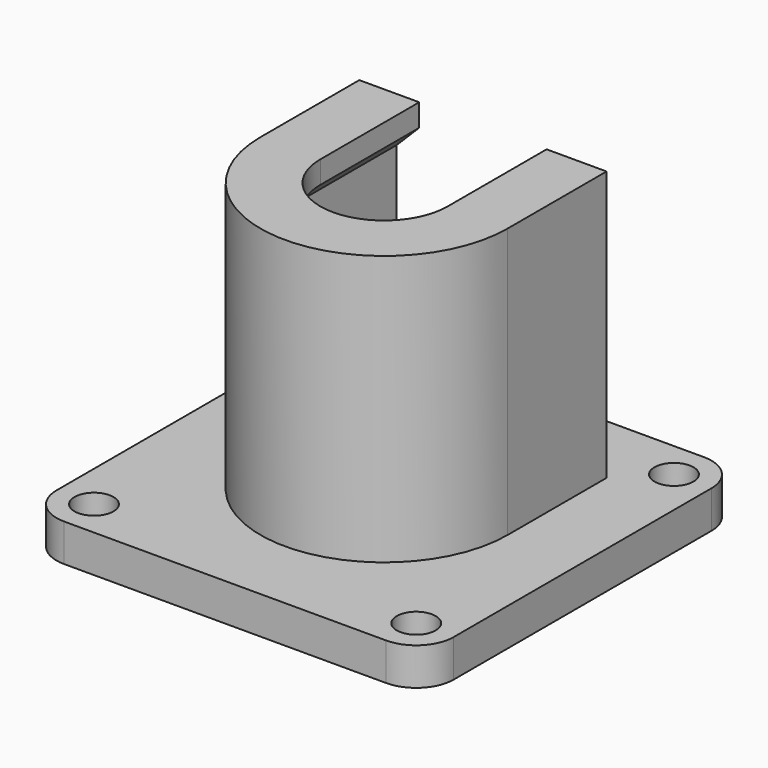
from build123d import *

# Parameters (mm, degrees)
F0_R     = 2.6
F1_DEPTH = 5
F3_DEPTH = 36
F6_DEPTH = 3
F9_DEPTH = 3
F10_SIZE = 2.99999


# Not quite as in the source:
# - a fillet or chamfer is up to 0.001 mm smaller than in the source, because OpenCascade refuses the exact size


with BuildPart() as f1:
    # F0 (on Top) → F1 (new body)
    with BuildSketch(Plane.XY):
        with BuildLine():
            Line((21.5, 26.5), (-21.5, 26.5))
            ThreePointArc((-21.5, 26.5), (-17.9644660941, 25.0355339059), (-16.5, 21.5))
            ThreePointArc((-16.5, 21.5), (-21.5, 16.5), (-26.5, 21.5))
            Line((-26.5, 21.5), (-26.5, -21.5))
            ThreePointArc((-26.5, -21.5), (-21.5, -16.5), (-16.5, -21.5))
            ThreePointArc((-16.5, -21.5), (-17.9644660941, -25.0355339059), (-21.5, -26.5))
            Line((-21.5, -26.5), (21.5, -26.5))
            ThreePointArc((21.5, -26.5), (17.9644660941, -17.9644660941), (26.5, -21.5))
            Line((26.5, -21.5), (26.5, 21.5))
            ThreePointArc((26.5, 21.5), (17.9644660941, 17.9644660941), (21.5, 26.5))
        make_face()
        with BuildLine():
            Line((-11.5, 16.5), (-11.5, 0))
            ThreePointArc((-11.5, 0), (0, -11.5), (11.5, 0))
            Line((11.5, 0), (11.5, 16.5))
            Line((11.5, 16.5), (16.5, 16.5))
            Line((16.5, 16.5), (16.5, 0))
            ThreePointArc((16.5, 0), (0, -16.5), (-16.5, 0))
            Line((-16.5, 0), (-16.5, 16.5))
            Line((-16.5, 16.5), (-11.5, 16.5))
        make_face(mode=Mode.SUBTRACT)
        with BuildLine():
            ThreePointArc((11.5, 0), (0, -11.5), (-11.5, 0))
            Line((-11.5, 0), (-11.5, 16.5))
            Line((-11.5, 16.5), (-16.5, 16.5))
            Line((-16.5, 16.5), (-16.5, 0))
            ThreePointArc((-16.5, 0), (0, -16.5), (16.5, 0))
            Line((16.5, 0), (16.5, 16.5))
            Line((16.5, 16.5), (11.5, 16.5))
            Line((11.5, 16.5), (11.5, 0))
        make_face()
        with BuildLine():
            ThreePointArc((-16.5, 21.5), (-17.9644660941, 25.0355339059), (-21.5, 26.5))
            ThreePointArc((-21.5, 26.5), (-25.0355339059, 25.0355339059), (-26.5, 21.5))
            ThreePointArc((-26.5, 21.5), (-21.5, 16.5), (-16.5, 21.5))
        make_face()
        with Locations((-21.5, 21.5)):
            Circle(F0_R, mode=Mode.SUBTRACT)
        with BuildLine():
            ThreePointArc((-16.5, -21.5), (-21.5, -16.5), (-26.5, -21.5))
            ThreePointArc((-26.5, -21.5), (-25.0355339059, -25.0355339059), (-21.5, -26.5))
            ThreePointArc((-21.5, -26.5), (-17.9644660941, -25.0355339059), (-16.5, -21.5))
        make_face()
        with Locations((-21.5, -21.5)):
            Circle(F0_R, mode=Mode.SUBTRACT)
        with BuildLine():
            ThreePointArc((21.5, -26.5), (25.0355339059, -25.0355339059), (26.5, -21.5))
            ThreePointArc((26.5, -21.5), (17.9644660941, -17.9644660941), (21.5, -26.5))
        make_face()
        with Locations((21.5, -21.5)):
            Circle(F0_R, mode=Mode.SUBTRACT)
        with BuildLine():
            ThreePointArc((26.5, 21.5), (25.0355339059, 25.0355339059), (21.5, 26.5))
            ThreePointArc((21.5, 26.5), (17.9644660941, 17.9644660941), (26.5, 21.5))
        make_face()
        with Locations((21.5, 21.5)):
            Circle(F0_R, mode=Mode.SUBTRACT)
    extrude(amount=F1_DEPTH)

    # F2 (on face) → F3 (join)
    with BuildSketch(Plane.XY.offset(5)):
        with BuildLine():
            ThreePointArc((11.5, 0), (0, -11.5), (-11.5, 0))
            Line((-11.5, 0), (-11.5, 16.5))
            Line((-11.5, 16.5), (-16.5, 16.5))
            Line((-16.5, 16.5), (-16.5, 0))
            ThreePointArc((-16.5, 0), (0, -16.5), (16.5, 0))
            Line((16.5, 0), (16.5, 16.5))
            Line((16.5, 16.5), (11.5, 16.5))
            Line((11.5, 16.5), (11.5, 0))
        make_face()
    extrude(amount=F3_DEPTH)

    # F5 (on offset) → F6 (join)
    with BuildSketch(Plane.XY.offset(15)):
        with BuildLine():
            Line((-11.5, 16.5), (-11.5, 0))
            ThreePointArc((-11.5, 0), (0, -11.5), (11.5, 0))
            Line((11.5, 0), (11.5, 16.5))
            Line((11.5, 16.5), (8.5, 16.5))
            Line((8.5, 16.5), (8.5, 0))
            ThreePointArc((8.5, 0), (0, -8.5), (-8.5, 0))
            Line((-8.5, 0), (-8.5, 16.5))
            Line((-8.5, 16.5), (-11.5, 16.5))
        make_face()
    extrude(amount=F6_DEPTH)

    # F8 (on offset) → F9 (join)
    with BuildSketch(Plane.XY.offset(38)):
        with BuildLine():
            Line((-11.5, 16.5), (-11.5, 0))
            ThreePointArc((-11.5, 0), (0, -11.5), (11.5, 0))
            Line((11.5, 0), (11.5, 16.5))
            Line((11.5, 16.5), (8.5, 16.5))
            Line((8.5, 16.5), (8.5, 0))
            ThreePointArc((8.5, 0), (0, -8.5), (-8.5, 0))
            Line((-8.5, 0), (-8.5, 16.5))
            Line((-8.5, 16.5), (-11.5, 16.5))
        make_face()
    extrude(amount=F9_DEPTH)

    # F10 (size 3 in the source; OpenCascade refuses exactly that, so slightly less here)
    f10_edges = [f1.edges().sort_by_distance(p)[0] for p in [
        (-11.5, 8.25, 38),
        (-11.5, 8.25, 15),
    ]]
    chamfer(f10_edges, length=F10_SIZE)


solid = f1.part
